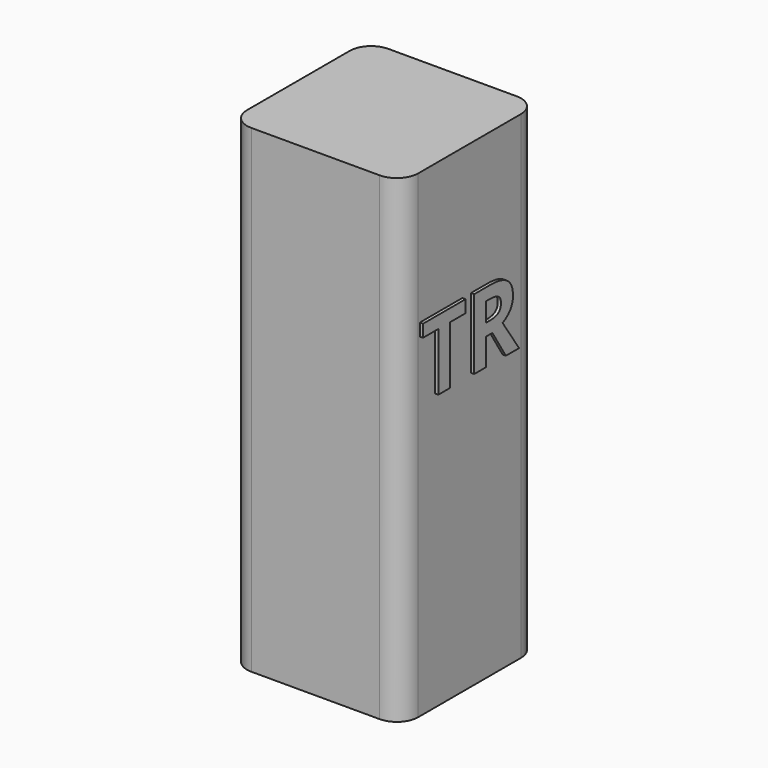
from build123d import *

# Parameters (mm, degrees)
F0_W         = 16
F0_H         = 16
F1_DEPTH     = 44.74
F2_R         = 2
F3_TEXT_SIZE = 9.2020129403
F4_DEPTH     = 0.3


# Not quite as in the source:
# - Text() gives the source's letters only with a copy of the font that has no kerning and outlines rounded to 1/6400 em; it was checked with that copy


with BuildPart() as f1:
    # F0 (on Top) → F1 (new body)
    with BuildSketch(Plane.XY):
        with Locations((8, 8)):
            Rectangle(F0_W, F0_H)
    extrude(amount=F1_DEPTH)

    # F2
    f2_edges = [f1.edges().sort_by_distance(p)[0] for p in [
        (16, 0, 22.37),
        (0, 0, 22.37),
        (16, 16, 22.37),
        (0, 16, 22.37),
    ]]
    fillet(f2_edges, radius=F2_R)

    # F3 (on face) → F4 (join)
    with BuildSketch(Plane.YZ.offset(16)):
        with Locations((2, 25.8236384533)):
            Text('TR', F3_TEXT_SIZE, font='Open Sans', font_style=FontStyle.BOLD, text_align=(TextAlign.LEFT, TextAlign.BOTTOM))
    extrude(amount=F4_DEPTH)


solid = f1.part
